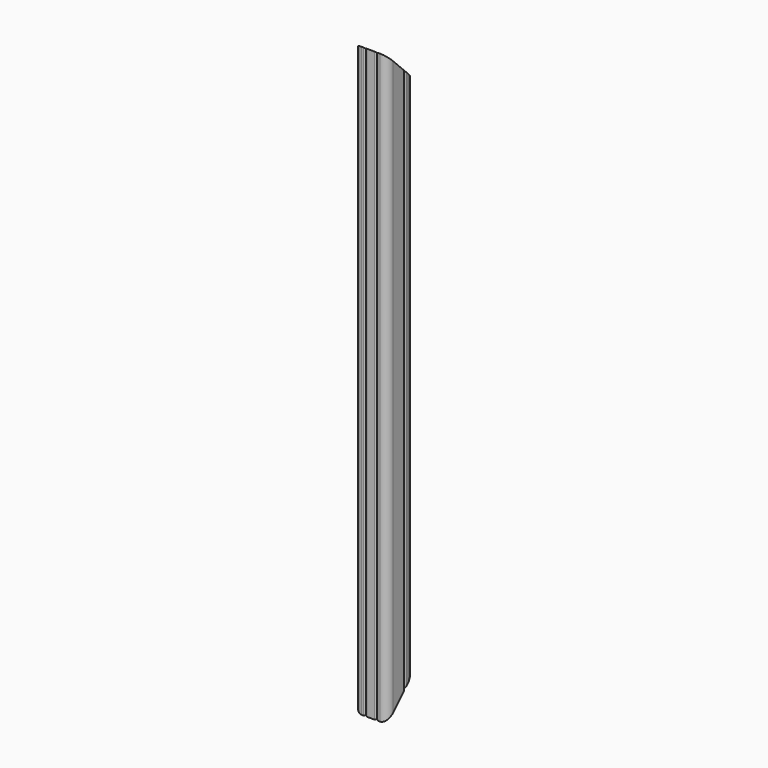
from build123d import *

# Parameters (mm, degrees)
F1_DEPTH = 1016
F3_DEPTH = 57.151


# Not quite as in the source:
# - ends of sketch curves that miss each other by under 0.0002 mm in the source are joined


with BuildPart() as f1:
    # F0 (on Top) → F1 (new body)
    with BuildSketch(Plane.XY):
        with BuildLine():
            ThreePointArc((0, 12.7), (3.7197438789, 3.7197438789), (12.7, 0))
            Line((12.7, 0), (15.9004, 0))
            ThreePointArc((15.9004, 0), (18.127503518, 0.922496482), (19.05, 3.1496))
            Line((19.05, 3.1496), (19.05, 34.9504))
            ThreePointArc((19.05, 34.9504), (18.127503518, 37.177503518), (15.9004, 38.1))
            Line((15.9004, 38.1), (3.1496, 38.1))
            ThreePointArc((3.1496, 38.1), (0.922496482, 37.177503518), (0, 34.9504))
            Line((0, 34.9504), (0, 12.7))
        make_face()
        with BuildLine():
            Line((19.05, 34.9504), (19.05, 3.1496))
            ThreePointArc((19.05, 3.1496), (19.972496482, 0.922496482), (22.1996, 0))
            Line((22.1996, 0), (34.9504, 0))
            ThreePointArc((34.9504, 0), (37.177503518, 0.922496482), (38.1, 3.1496))
            Line((38.1, 3.1496), (38.1, 34.9504))
            ThreePointArc((38.1, 34.9504), (37.177503518, 37.177503518), (34.9504, 38.1))
            Line((34.9504, 38.1), (22.1996, 38.1))
            ThreePointArc((22.1996, 38.1), (19.972496482, 37.177503518), (19.05, 34.9504))
        make_face()
        with BuildLine():
            Line((38.1, 34.9504), (38.1, 3.1496))
            ThreePointArc((38.1, 3.1496), (39.022496482, 0.922496482), (41.2496, 0))
            Line((41.2496, 0), (44.45, 0))
            ThreePointArc((44.45, 0), (53.4302561211, 3.7197438789), (57.15, 12.7))
            Line((57.15, 12.7), (57.15, 34.9504))
            ThreePointArc((57.15, 34.9504), (56.227503518, 37.177503518), (54.0004, 38.1))
            Line((54.0004, 38.1), (41.2496, 38.1))
            ThreePointArc((41.2496, 38.1), (39.022496482, 37.177503518), (38.1, 34.9504))
        make_face()
        with BuildLine():
            ThreePointArc((19.0499988437, 41.2496), (19.9724953256, 39.022496482), (22.1995988437, 38.1))
            Line((22.1995988437, 38.1), (34.9504, 38.1))
            Line((34.9504, 38.1), (41.2496, 38.1))
            Line((41.2496, 38.1), (54.0004, 38.1))
            ThreePointArc((54.0004, 38.1), (56.2275023617, 39.022496482), (57.1499988437, 41.2496))
            Line((57.1499988437, 41.2496), (57.1499988437, 44.45))
            ThreePointArc((57.1499988437, 44.45), (53.4302549647, 53.4302561211), (44.4499988437, 57.15))
            Line((44.4499988437, 57.15), (22.1995988437, 57.15))
            ThreePointArc((22.1995988437, 57.15), (19.9724953256, 56.227503518), (19.0499988437, 54.0004))
            Line((19.0499988437, 54.0004), (19.0499988437, 41.2496))
        make_face()
    extrude(amount=F1_DEPTH)

    # F2 (on face) → F3 (cut, through all)
    with BuildSketch(Plane.YZ.offset(57.15)):
        Polygon((57.15, 0), (57.15, 57.15), (0, 0), (12.7, 0), align=None)
        Polygon((12.7, 1016), (0, 1016), (57.15, 958.85), (57.15, 1016), align=None)
    extrude(amount=-F3_DEPTH, mode=Mode.SUBTRACT)


solid = f1.part
